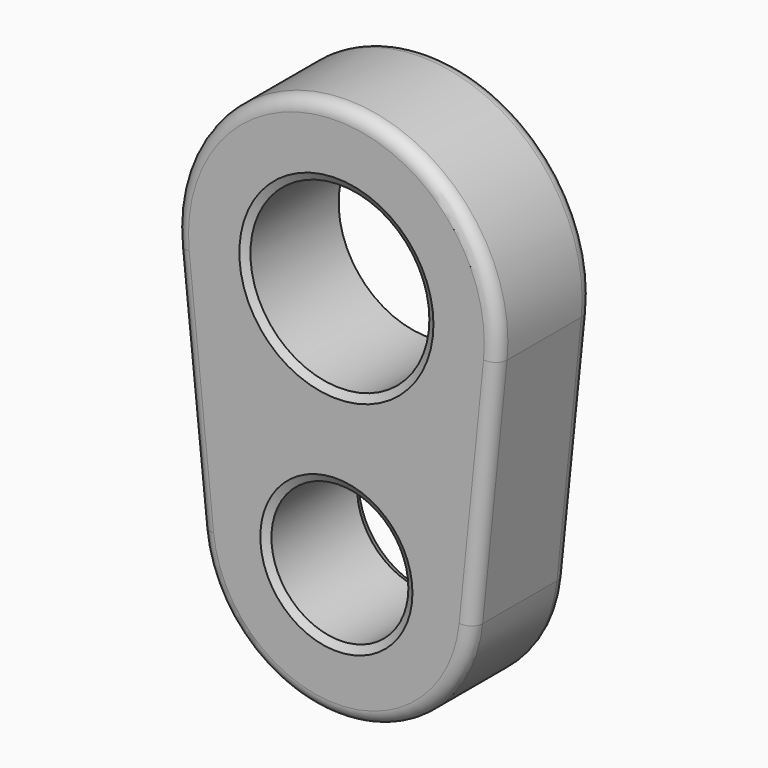
from build123d import *

# Parameters (mm, degrees)
F1_DEPTH    = 3.4544
F2_R        = 2.59715
F2_R_2      = 1.98755
F3_DEPTH    = 3.4554
F4_C1_SIZE2 = 0.127
F4_C1_SIZE  = 0.2199704526
F4_C2_SIZE2 = 0.127
F4_C2_SIZE  = 0.2199704526
F4_C3_SIZE2 = 0.127
F4_C3_SIZE  = 0.2199704526
F4_C4_SIZE2 = 0.127
F4_C4_SIZE  = 0.2199704526
F5_R        = 0.381


with BuildPart() as f1:
    # F0 (on Front) → F1 (new body)
    with BuildSketch(Plane.XZ):
        with BuildLine():
            Line((3.9421045586, -3.9184314079), (4.6496617871, 3.0454783394))
            ThreePointArc((4.6496617871, 3.0454783394), (0, 8.1915), (-4.6496617871, 3.0454783394))
            Line((-4.6496617871, 3.0454783394), (-3.9421045586, -3.9184314079))
            ThreePointArc((-3.9421045586, -3.9184314079), (0, -7.4803), (3.9421045586, -3.9184314079))
        make_face()
    extrude(amount=-F1_DEPTH)

    # F2 (on face) → F3 (cut, through all)
    with BuildSketch(Plane.XZ):
        with Locations((0, 3.5179)):
            Circle(F2_R)
        with Locations((0, -3.5433)):
            Circle(F2_R_2)
    extrude(amount=-F3_DEPTH, mode=Mode.SUBTRACT)

    # F4: chamfer of 0.127 x 0.2199704526 on 4 edges, made by hand

    # F4_c1
    f4_c1_edges = [f1.edges().sort_by_distance(p)[0] for p in [
        (-1.98755, 0, -3.5433),
    ]]
    f4_c1_side = f1.faces().sort_by_distance((-1.99009, 0, -3.5433))[0]
    chamfer(f4_c1_edges, length=F4_C1_SIZE, length2=F4_C1_SIZE2, reference=f4_c1_side)

    # F4_c2
    f4_c2_edges = [f1.edges().sort_by_distance(p)[0] for p in [
        (-2.59715, 0, 3.5179),
    ]]
    f4_c2_side = f1.faces().sort_by_distance((-2.59969, 0, 3.5179))[0]
    chamfer(f4_c2_edges, length=F4_C2_SIZE, length2=F4_C2_SIZE2, reference=f4_c2_side)

    # F4_c3
    f4_c3_edges = [f1.edges().sort_by_distance(p)[0] for p in [
        (-1.98755, 3.4544, -3.5433),
    ]]
    f4_c3_side = f1.faces().sort_by_distance((-1.98755, 3.45186, -3.5433))[0]
    chamfer(f4_c3_edges, length=F4_C3_SIZE, length2=F4_C3_SIZE2, reference=f4_c3_side)

    # F4_c4
    f4_c4_edges = [f1.edges().sort_by_distance(p)[0] for p in [
        (-2.59715, 3.4544, 3.5179),
    ]]
    f4_c4_side = f1.faces().sort_by_distance((-2.59969, 3.4544, 3.5179))[0]
    chamfer(f4_c4_edges, length=F4_C4_SIZE, length2=F4_C4_SIZE2, reference=f4_c4_side)

    # F5
    f5_edges = [f1.edges().sort_by_distance(p)[0] for p in [
        (0, 0, -7.4803),
        (0, 3.4544, -7.4803),
        (4.295883, 3.4544, -0.436477),
        (0, 3.4544, 8.1915),
        (-4.295883, 3.4544, -0.436477),
        (4.295883, 0, -0.436477),
        (0, 0, 8.1915),
        (-4.295883, 0, -0.436477),
    ]]
    fillet(f5_edges, radius=F5_R)


solid = f1.part
